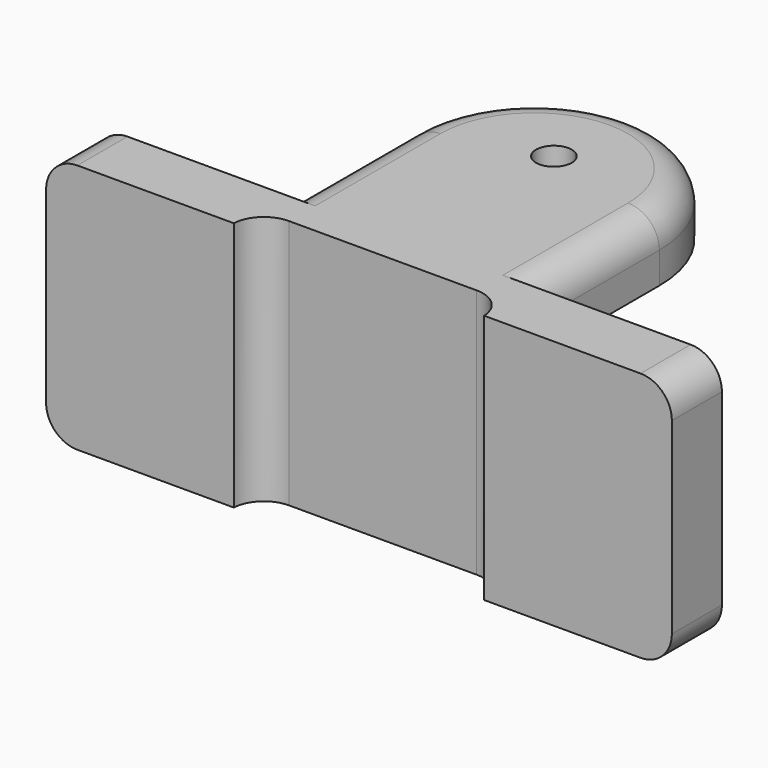
from build123d import *

# Parameters (mm, degrees)
F0_W          = 100
F0_H          = 40
F1_DEPTH      = 10
F3_DEPTH      = 10
F4_W          = 40
F4_H          = 3
F5_DEPTH      = 174
F6_W          = 40
F6_H          = 4.7629310191
F7_DEPTH      = 40.001
F8_R          = 2.85
F9_DEPTH      = 40.001
F10_T1_DEPTH  = 40
F10_T3_DEPTH  = 40
F10_T5_DEPTH  = 35
F10_T7_DEPTH  = 35
F10_T9_DEPTH  = 35
F10_T11_DEPTH = 35
F10_T13_DEPTH = 25
F10_T16_ANGLE = 180


# Not quite as in the source:
# - a fillet or chamfer that OpenCascade refuses, or shapes differently, is made with other operations: its cross-section is extruded or revolved along the edge and cut away or added
# - two fillets or chamfers of one size are made in one step
# - an extrude ends at something that could not be found from the text; its depth is read off the source's solid


with BuildPart() as f1:
    # F0 (on Front) → F1 (new body)
    with BuildSketch(Plane.XZ):
        with Locations((-50, 20)):
            Rectangle(F0_W, F0_H)
    extrude(amount=F1_DEPTH)

    # F2 (on face) → F3 (join)
    with BuildSketch(Plane.XY.offset(40)):
        with BuildLine():
            Line((-70, 25), (-70, 0))
            Line((-70, 0), (-70, -10))
            Line((-70, -10), (-30, -10))
            Line((-30, -10), (-30, 0))
            Line((-30, 0), (-30, 25))
            ThreePointArc((-30, 25), (-50, 45), (-70, 25))
        make_face()
        with BuildLine():
            Line((-70, 25), (-70, 0))
            Line((-70, 0), (-30, 0))
            Line((-30, 0), (-30, 25))
            ThreePointArc((-30, 25), (-50, 45), (-70, 25))
        make_face()
    extrude(amount=-F3_DEPTH)

    # F4 (on face) → F5 (cut, through all)
    with BuildSketch(Plane.XY.offset(40)):
        with Locations((-50, -8.5)):
            Rectangle(F4_W, F4_H)
    extrude(amount=F5_DEPTH, mode=Mode.SUBTRACT)

    # F6 (on face) → F7 (cut, through all)
    with BuildSketch(Plane.XY.offset(40)):
        with Locations((-50, -7.6185344905)):
            Rectangle(F6_W, F6_H)
    extrude(amount=-F7_DEPTH, mode=Mode.SUBTRACT)

    # F8 (on face) → F9 (cut, through all)
    with BuildSketch(Plane.XY.offset(40)):
        with Locations((-50.1293092966, 29.0948301554)):
            Circle(F8_R)
    extrude(amount=-F9_DEPTH, mode=Mode.SUBTRACT)

    # F10: fillet of radius 5 on 9 edges, made by hand

    # F10_s2 → F10_t1 (join)
    with BuildSketch(Plane.XY):
        with BuildLine():
            ThreePointArc((-30, -10), (-31.543677094, -6.6186891705), (-34.9943766676, -5.2370689809))
            Line((-34.9943766676, -5.2370689809), (-30, -5.2370689809))
            Line((-30, -5.2370689809), (-30, -10))
        make_face()
    extrude(amount=F10_T1_DEPTH)

    # F10_s4 → F10_t3 (join)
    with BuildSketch(Plane.XY):
        with BuildLine():
            ThreePointArc((-65.0056233324, -5.2370689809), (-68.456322906, -6.6186891705), (-70, -10))
            Line((-70, -10), (-70, -5.2370689809))
            Line((-70, -5.2370689809), (-65.0056233324, -5.2370689809))
        make_face()
    extrude(amount=F10_T3_DEPTH)

    # F10_s6 → F10_t5 (cut)
    with BuildSketch(Plane.XZ.offset(-12.5)):
        with BuildLine():
            ThreePointArc((-5, 0), (-1.4644660941, 1.4644660941), (0, 5))
            Line((0, 5), (0, 0))
            Line((0, 0), (-5, 0))
        make_face()
    extrude(amount=F10_T5_DEPTH, mode=Mode.SUBTRACT)

    # F10_s8 → F10_t7 (cut)
    with BuildSketch(Plane.XZ.offset(-12.5)):
        with BuildLine():
            ThreePointArc((-95, 0), (-98.5355339059, 1.4644660941), (-100, 5))
            Line((-100, 5), (-100, 0))
            Line((-100, 0), (-95, 0))
        make_face()
    extrude(amount=F10_T7_DEPTH, mode=Mode.SUBTRACT)

    # F10_s10 → F10_t9 (cut)
    with BuildSketch(Plane.XZ.offset(-12.5)):
        with BuildLine():
            ThreePointArc((-5, 40), (-1.4644660941, 38.5355339059), (0, 35))
            Line((0, 35), (0, 40))
            Line((0, 40), (-5, 40))
        make_face()
    extrude(amount=F10_T9_DEPTH, mode=Mode.SUBTRACT)

    # F10_s12 → F10_t11 (cut)
    with BuildSketch(Plane.XZ.offset(-12.5)):
        with BuildLine():
            ThreePointArc((-95, 40), (-98.5355339059, 38.5355339059), (-100, 35))
            Line((-100, 35), (-100, 40))
            Line((-100, 40), (-95, 40))
        make_face()
    extrude(amount=F10_T11_DEPTH, mode=Mode.SUBTRACT)

    # F10_s14 → F10_t13 (cut)
    with BuildSketch(Plane.XZ.offset(-25)):
        with BuildLine():
            ThreePointArc((-70, 35), (-68.5355339059, 38.5355339059), (-65, 40))
            Line((-65, 40), (-70, 40))
            Line((-70, 40), (-70, 35))
        make_face()
        with BuildLine():
            ThreePointArc((-30, 35), (-31.4644660941, 38.5355339059), (-35, 40))
            Line((-35, 40), (-30, 40))
            Line((-30, 40), (-30, 35))
        make_face()
    extrude(amount=F10_T13_DEPTH, mode=Mode.SUBTRACT)

    # F10_s15 → F10_t16 (revolve, cut)
    with BuildSketch(Plane.XZ.offset(-25)):
        with BuildLine():
            ThreePointArc((-35, 40), (-31.4644660941, 38.5355339059), (-30, 35))
            Line((-30, 35), (-30, 40))
            Line((-30, 40), (-35, 40))
        make_face()
    revolve(axis=Axis((-50, 25, 40), (0, 0, 1)), revolution_arc=F10_T16_ANGLE, mode=Mode.SUBTRACT)


solid = f1.part
